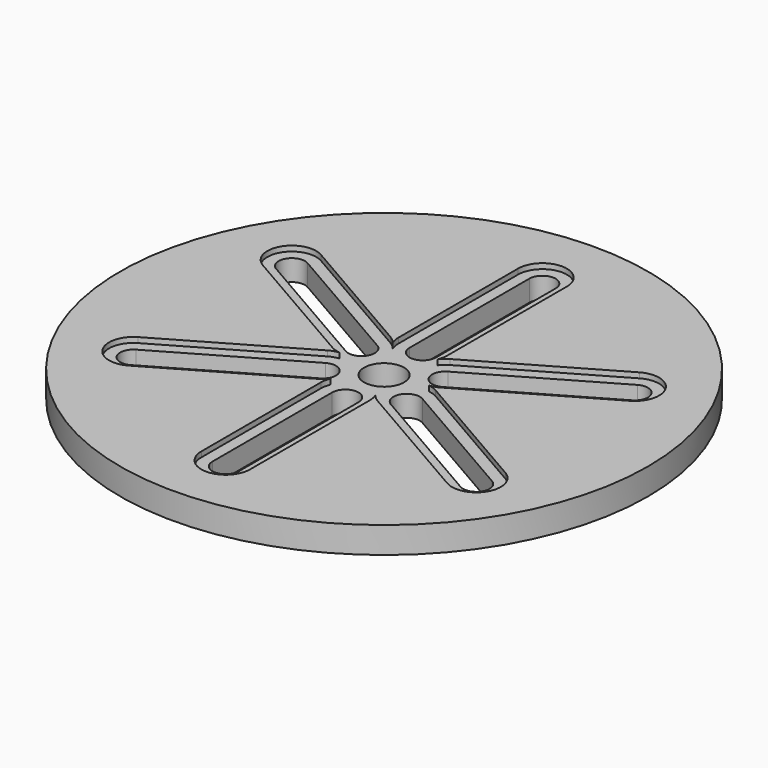
from build123d import *

# Parameters (mm, degrees)
F0_R            = 150
F1_DEPTH        = 15
F3_DEPTH        = 15.001
F3_COPIES_COUNT = 6
F5_DEPTH        = 3
F5_COPIES_COUNT = 6
F6_R            = 25
F6_R_2          = 11.35
F7_DEPTH        = 3
F8_DEPTH        = 15.001


# Not quite as in the source:
# - an extrude ends at something that could not be found from the text; its depth is read off the source's solid
# - a pattern or mirror of a feature is missing from the dataset's text; its kind, count and spacing are read off the source's solid


with BuildPart() as f1:
    # F0 (on Top) → F1 (new body)
    with BuildSketch(Plane.XY):
        Circle(F0_R)
    extrude(amount=F1_DEPTH)

    # F2 (on face) → F3 (cut, through all)
    with BuildSketch(Plane.XY.offset(15)):
        with BuildLine():
            ThreePointArc((0, 120), (-5.3033008589, 117.8033008589), (-7.5, 112.5))
            Line((-7.5, 112.5), (-7.5, 27.5))
            ThreePointArc((-7.5, 27.5), (-5.3033008589, 22.1966991411), (0, 20))
            Line((0, 20), (0, 120))
        make_face()
        with BuildLine():
            ThreePointArc((7.5, 112.5), (5.3033008589, 117.8033008589), (0, 120))
            Line((0, 120), (0, 20))
            ThreePointArc((0, 20), (5.3033008589, 22.1966991411), (7.5, 27.5))
            Line((7.5, 27.5), (7.5, 112.5))
        make_face()
    f3 = extrude(amount=-F3_DEPTH, mode=Mode.SUBTRACT)

    # F3_copies: F3 ×6 about axis
    f3_copies_axis = Axis((0, 0, 0), (0, 0, 1))
    for i in range(1, F3_COPIES_COUNT):
        add(f3.rotate(f3_copies_axis, i * 360 / F3_COPIES_COUNT), mode=Mode.SUBTRACT)

    # F4 (on face) → F5 (cut)
    with BuildSketch(Plane.XY.offset(15)):
        with BuildLine():
            Line((13.85, 27.5), (13.85, 112.5))
            ThreePointArc((13.85, 112.5), (0, 126.35), (-13.85, 112.5))
            Line((-13.85, 112.5), (-13.85, 27.5))
            ThreePointArc((-13.85, 27.5), (0, 13.65), (13.85, 27.5))
        make_face()
        with BuildLine():
            Line((7.5, 112.5), (7.5, 27.5))
            ThreePointArc((7.5, 27.5), (0, 20), (-7.5, 27.5))
            Line((-7.5, 27.5), (-7.5, 112.5))
            ThreePointArc((-7.5, 112.5), (0, 120), (7.5, 112.5))
        make_face(mode=Mode.SUBTRACT)
    f5 = extrude(amount=-F5_DEPTH, mode=Mode.SUBTRACT)

    # F5_copies: F5 ×6 about axis
    f5_copies_axis = Axis((0, 0, 0), (0, 0, 1))
    for i in range(1, F5_COPIES_COUNT):
        add(f5.rotate(f5_copies_axis, i * 360 / F5_COPIES_COUNT), mode=Mode.SUBTRACT)

    # F6 (on face) → F7 (cut, through all)
    with BuildSketch(Plane.XY.offset(15)):
        Circle(F6_R)
        with BuildLine():
            ThreePointArc((11.0771869157, 19.186250543), (11.8212467617, 6.825), (22.1543738315, 0))
            ThreePointArc((22.1543738315, 0), (11.8212467617, -6.825), (11.0771869157, -19.186250543))
            ThreePointArc((11.0771869157, -19.186250543), (0, -13.65), (-11.0771869157, -19.186250543))
            ThreePointArc((-11.0771869157, -19.186250543), (-11.8212467617, -6.825), (-22.1543738315, 0))
            ThreePointArc((-22.1543738315, 0), (-11.8212467617, 6.825), (-11.0771869157, 19.186250543))
            ThreePointArc((-11.0771869157, 19.186250543), (0, 13.65), (11.0771869157, 19.186250543))
        make_face(mode=Mode.SUBTRACT)
        with BuildLine():
            ThreePointArc((11.0771869157, -19.186250543), (11.8212467617, -6.825), (22.1543738315, 0))
            ThreePointArc((22.1543738315, 0), (11.8212467617, 6.825), (11.0771869157, 19.186250543))
            ThreePointArc((11.0771869157, 19.186250543), (0, 13.65), (-11.0771869157, 19.186250543))
            ThreePointArc((-11.0771869157, 19.186250543), (-11.8212467617, 6.825), (-22.1543738315, 0))
            ThreePointArc((-22.1543738315, 0), (-11.8212467617, -6.825), (-11.0771869157, -19.186250543))
            ThreePointArc((-11.0771869157, -19.186250543), (0, -13.65), (11.0771869157, -19.186250543))
        make_face()
        Circle(F6_R_2, mode=Mode.SUBTRACT)
        Circle(F6_R_2)
    extrude(amount=-F7_DEPTH, mode=Mode.SUBTRACT)

    # F6 (on face) → F8 (cut, through all)
    with BuildSketch(Plane.XY.offset(15)):
        Circle(F6_R_2)
    extrude(amount=-F8_DEPTH, mode=Mode.SUBTRACT)


solid = f1.part
